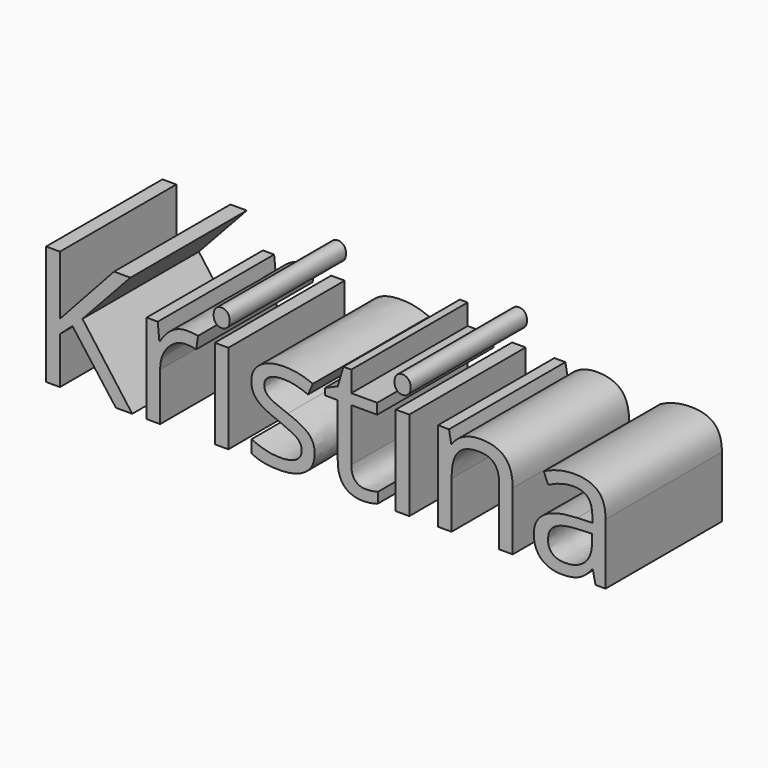
from build123d import *

# Parameters (mm, degrees)
F0_TEXT_SIZE = 29.1723861463
F1_DEPTH     = 25.4


# Not quite as in the source:
# - Text() gives the source's letters only with a copy of the font that has no kerning and outlines rounded to 1/6400 em; it was checked with that copy


with BuildPart() as f1:
    # F0 (on Front) → F1 (new body)
    with BuildSketch(Plane.XZ):
        with Locations((-49.6307164431, 8.9775621891)):
            Text('Kristina', F0_TEXT_SIZE, font='Open Sans', text_align=(TextAlign.LEFT, TextAlign.BOTTOM))
    extrude(amount=F1_DEPTH)


solid = f1.part
